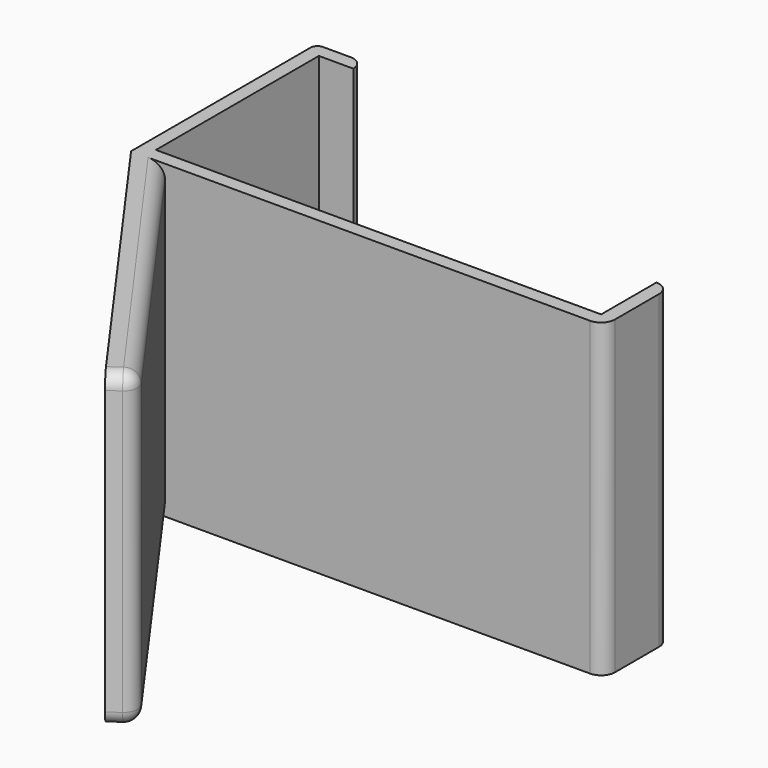
from build123d import *

# Parameters (mm, degrees)
F1_DEPTH = 45
F2_R     = 1.99999
F4_R     = 1
F3_R     = 5
F5_DEPTH = 3.1


# Not quite as in the source:
# - a fillet or chamfer is up to 0.001 mm smaller than in the source, because OpenCascade refuses the exact size
# - a feature names something its author has since deleted; it is built from what else it names


with BuildPart() as f1:
    # F0 (on Top) → F1 (new body)
    with BuildSketch(Plane.XY):
        Polygon((30.2546076554, -42.2925373514), (0, 0), (63.5818746515, 0), (63.5818746515, 12), (61.5818746515, 12), (61.5818746515, 2), (-2.9181253485, 2), (-2.9181253485, 31.5), (2.0818746515, 31.5), (2.0818746515, 33.5), (-4.9181253485, 33.5), (-4.9181253485, 31.5), (-4.9181253485, 0), (27.0013355514, -44.6198148634), align=None)
    extrude(amount=F1_DEPTH)

    # F2 (radius 2 in the source; OpenCascade refuses exactly that, so slightly less here)
    f2_edges = [f1.edges().sort_by_distance(p)[0] for p in [
        (63.581875, 0, 22.5),
        (63.581875, 12, 22.5),
        (30.254608, -42.292537, 22.5),
        (28.627972, -43.456176, 45),
        (28.627972, -43.456176, 0),
        (15.127304, -21.146269, 45),
        (15.127304, -21.146269, 0),
        (2.081875, 33.5, 22.5),
    ]]
    fillet(f2_edges, radius=F2_R)

    # F4
    f4_edges = [f1.edges().sort_by_distance(p)[0] for p in [
        (-4.918125, 33.5, 22.5),
    ]]
    fillet(f4_edges, radius=F4_R)

    # F3 (on face) → F5 (cut)
    with BuildSketch(Plane(origin=(-3.253272104, -2.327277512, 0), x_dir=(0.581819378, -0.813318026, 0), z_dir=(-0.813318026, -0.581819378, 0))):
        with Locations((22.1385393689, 12.5)):
            Circle(F3_R)
        with Locations((22.1385393689, 32.5)):
            Circle(F3_R)
    extrude(amount=-F5_DEPTH, mode=Mode.SUBTRACT)


solid = f1.part
